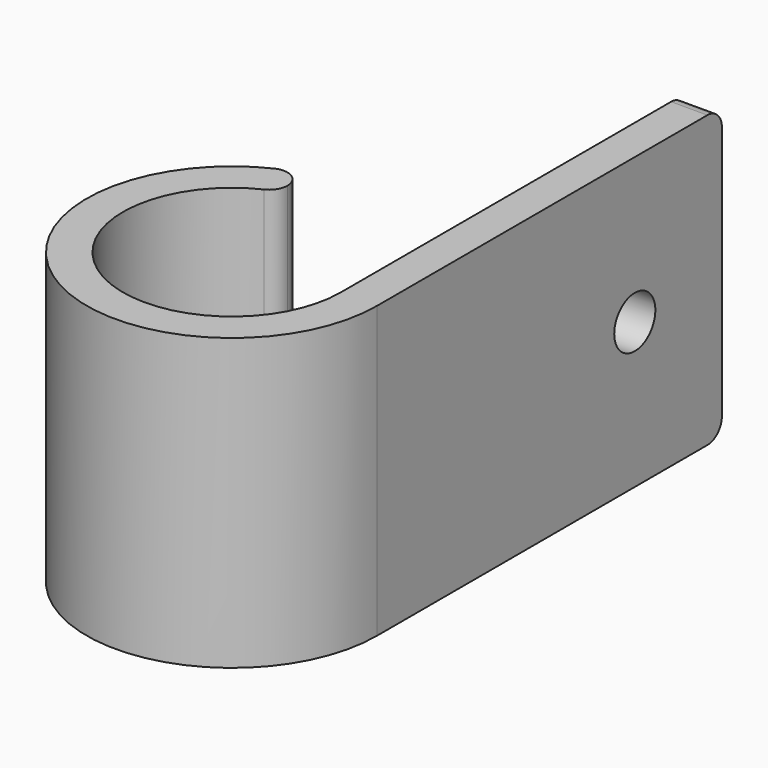
from build123d import *

# Parameters (mm, degrees)
F1_DEPTH = 12.7
F2_R     = 1.58749
F3_R     = 1.5875
F5_D     = 4.4958


# Not quite as in the source:
# - a fillet or chamfer is up to 0.001 mm smaller than in the source, because OpenCascade refuses the exact size


with BuildPart() as f1:
    # F0 (on Top) → F1 (new body, symmetric)
    with BuildSketch(Plane.XY):
        with BuildLine():
            Line((0, 37.6967221242), (0, 0))
            ThreePointArc((0, 0), (-15.024261314, -7.7771299333), (-12.7, 8.9802561211))
            Line((-12.7, 8.9802561211), (-12.7, 12.2967221242))
            ThreePointArc((-12.7, 12.2967221242), (-17.3021299333, -10.040231571), (3.175, 0))
            Line((3.175, 0), (3.175, 37.6967221242))
            Line((3.175, 37.6967221242), (0, 37.6967221242))
        make_face()
    extrude(amount=F1_DEPTH, both=True)

    # F2 (radius 1.5875 in the source; OpenCascade refuses exactly that, so slightly less here)
    f2_edges = [f1.edges().sort_by_distance(p)[0] for p in [
        (-12.7, 8.980256, 0),
        (-12.7, 12.296722, 0),
    ]]
    fillet(f2_edges, radius=F2_R)

    # F3
    f3_edges = [f1.edges().sort_by_distance(p)[0] for p in [
        (1.5875, 37.696722, 12.7),
        (1.5875, 37.696722, -12.7),
    ]]
    fillet(f3_edges, radius=F3_R)

    # F5 (through all)
    with Locations(Plane(origin=(0, 0, 0), x_dir=(0, 1, 0), z_dir=(-1, 0, 0))):
        with Locations((28.1717221242, 0)):
            Hole(F5_D / 2)


solid = f1.part
